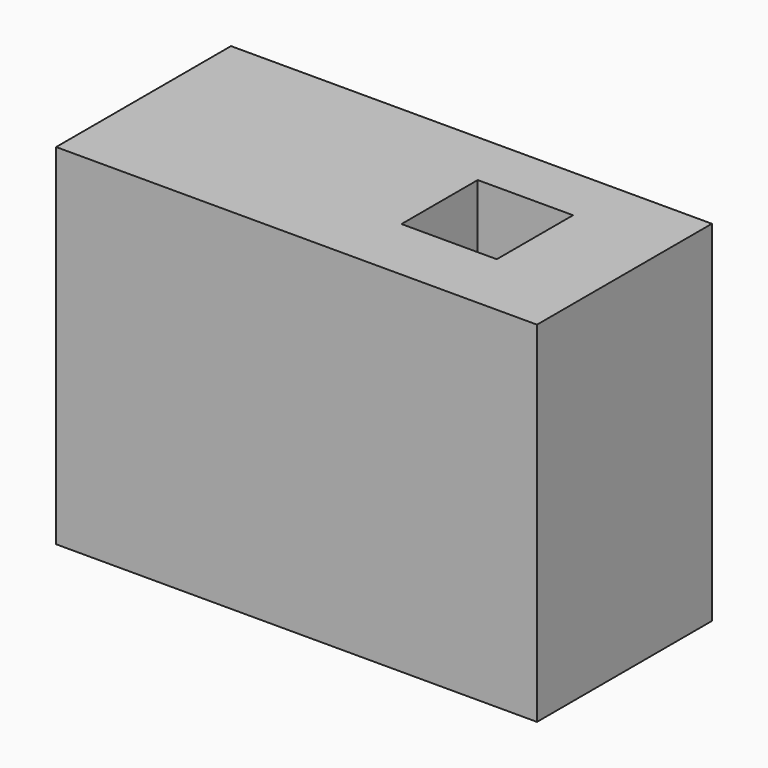
from build123d import *

# Parameters (mm, degrees)
F0_W     = 27.94
F0_H     = 20.32
F1_DEPTH = 12.7
F2_W     = 5.5372
F2_H     = 5.5372
F3_DEPTH = 18.542


# Not quite as in the source:
# - a feature names something its author has since deleted; it is built from what else it names


with BuildPart() as f1:
    # F0 (on Front) → F1 (new body)
    with BuildSketch(Plane.XZ):
        Rectangle(F0_W, F0_H)
    extrude(amount=F1_DEPTH)

    # F2 (on face) → F3 (cut)
    with BuildSketch(Plane.XY.offset(10.16)):
        with Locations((5.760986782, -6.0524168657)):
            Rectangle(F2_W, F2_H)
    extrude(amount=-F3_DEPTH, mode=Mode.SUBTRACT)


solid = f1.part
